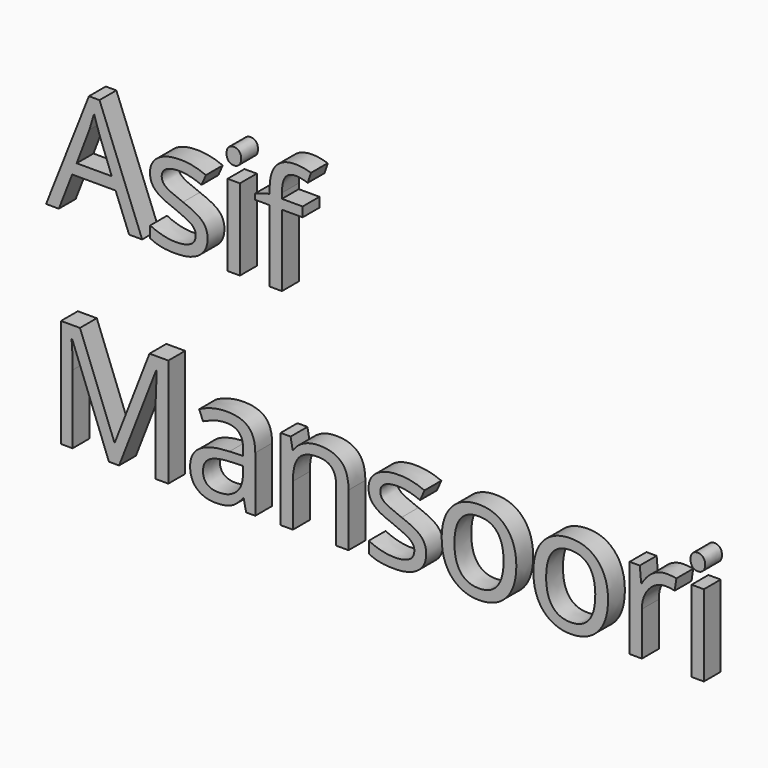
from build123d import *

# Parameters (mm, degrees)
F0_TEXT_SIZE = 91.6020013392
F1_DEPTH     = 12.7


# Not quite as in the source:
# - Text() gives the source's letters only with a copy of the font that has no kerning and outlines rounded to 1/6400 em; it was checked with that copy


with BuildPart() as f1:
    # F0 (on Front) → F1 (new body)
    with BuildSketch(Plane.XZ):
        with Locations((-68.8290446997, 0)):
            Text('Asif', F0_TEXT_SIZE, font='Open Sans', text_align=(TextAlign.LEFT, TextAlign.BOTTOM))
        with Locations((-68.8290446997, -124.5787218213)):
            Text('Mansoori', F0_TEXT_SIZE, font='Open Sans', text_align=(TextAlign.LEFT, TextAlign.BOTTOM))
    extrude(amount=F1_DEPTH)


solid = f1.part
